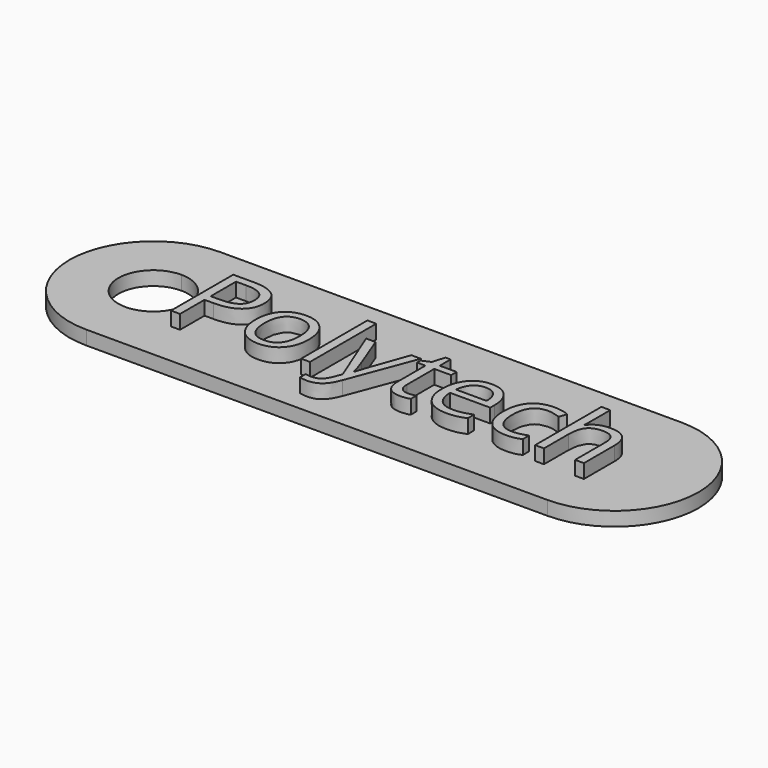
from build123d import *

# Parameters (mm, degrees)
F0_TEXT_SIZE = 7.7975032327
F1_DEPTH     = 2
F0_W         = 0.6323287778
F0_H         = 5.924884097
F2_DEPTH     = 1


# Not quite as in the source:
# - Text() gives the source's letters only with a copy of the font that has no kerning and outlines rounded to 1/6400 em; it was checked with that copy


with BuildPart() as f1:
    # F0 (on Top) → F1 (new body)
    with BuildSketch(Plane.XY):
        with Locations((-13.804265298, -2.749341398)):
            Text('Polytech', F0_TEXT_SIZE, font='Open Sans', text_align=(TextAlign.LEFT, TextAlign.BOTTOM))
    extrude(amount=F1_DEPTH)


with BuildPart() as f2:
    # F0 (on Top) → F2 (new body)
    with BuildSketch(Plane.XY):
        with BuildLine():
            Line((16.5, -0.0275254258), (16.5, 6))
            Line((16.5, 6), (-16.5, 6))
            Line((-16.5, 6), (-16.5, 2.5))
            ThreePointArc((-16.5, 2.5), (-14.732233047, 1.767766953), (-14, 0))
            ThreePointArc((-14, 0), (-14.732233047, -1.767766953), (-16.5, -2.5))
            Line((-16.5, -2.5), (-16.5, -6))
            Line((-16.5, -6), (16.5, -6))
            Line((16.5, -6), (16.5, -2.749341398))
            Line((16.5, -2.749341398), (15.8676712222, -2.749341398))
            Line((15.8676712222, -2.749341398), (15.8676712222, -0.0494559037))
            add(Edge.make_bspline(
                [(15.8676712222, -0.0494559037), (15.8676712222, 0.4598185262), (15.6355736651, 0.7114098415)],
                knots=[0, 0, 0, 1, 1, 1], degree=2))
            add(Edge.make_bspline(
                [(15.6355736651, 0.7114098415), (15.4034761079, 0.9630011567), (14.9076036367, 0.9630011567)],
                knots=[0, 0, 0, 1, 1, 1], degree=2))
            add(Edge.make_bspline(
                [(14.9076036367, 0.9630011567), (14.2496893014, 0.9630011567), (13.9469268712, 0.6048033519)],
                knots=[0, 0, 0, 1, 1, 1], degree=2))
            add(Edge.make_bspline(
                [(13.9469268712, 0.6048033519), (13.644164441, 0.2466055472), (13.644164441, -0.5672588527)],
                knots=[0, 0, 0, 1, 1, 1], degree=2))
            Line((13.644164441, -0.5672588527), (13.644164441, -2.749341398))
            Line((13.644164441, -2.749341398), (13.0118356632, -2.749341398))
            Line((13.0118356632, -2.749341398), (13.0118356632, 3.175542699))
            Line((13.0118356632, 3.175542699), (13.644164441, 3.175542699))
            Line((13.644164441, 3.175542699), (13.644164441, 1.3821169555))
            add(Edge.make_bspline(
                [(13.644164441, 1.3821169555), (13.644164441, 1.0580332273), (13.613705444, 0.8448202483)],
                knots=[0, 0, 0, 1, 1, 1], degree=2))
            Line((13.613705444, 0.8448202483), (13.6514746003, 0.8448202483))
            add(Edge.make_bspline(
                [(13.6514746003, 0.8448202483), (13.837883662, 1.1457551387), (14.182679508, 1.3187622417)],
                knots=[0, 0, 0, 1, 1, 1], degree=2))
            add(Edge.make_bspline(
                [(14.182679508, 1.3187622417), (14.5274753541, 1.4917693447), (14.9685216307, 1.4917693447)],
                knots=[0, 0, 0, 1, 1, 1], degree=2))
            add(Edge.make_bspline(
                [(14.9685216307, 1.4917693447), (15.7336516354, 1.4917693447), (16.1168258177, 1.1280889205)],
                knots=[0, 0, 0, 1, 1, 1], degree=2))
            add(Edge.make_bspline(
                [(16.1168258177, 1.1280889205), (16.5, 0.7644084962), (16.5, -0.0275254258)],
                knots=[0, 0, 0, 1, 1, 1], degree=2))
        make_face()
        with BuildLine():
            Line((-0.7361372239, -2.7724902357), (-2.4199105782, 1.4235411914))
            Line((-2.4199105782, 1.4235411914), (-1.741284125, 1.4235411914))
            Line((-1.741284125, 1.4235411914), (-0.8275142149, -0.9559156545))
            add(Edge.make_bspline(
                [(-0.8275142149, -0.9559156545), (-0.5277976844, -1.7709984143), (-0.4546960916, -2.1328512987)],
                knots=[0, 0, 0, 1, 1, 1], degree=2))
            Line((-0.4546960916, -2.1328512987), (-0.4242370946, -2.1328512987))
            add(Edge.make_bspline(
                [(-0.4242370946, -2.1328512987), (-0.3755026994, -1.9379137179), (-0.217115915, -1.4676268041)],
                knots=[0, 0, 0, 1, 1, 1], degree=2))
            add(Edge.make_bspline(
                [(-0.217115915, -1.4676268041), (-0.0587291306, -0.9973398904), (0.8172716232, 1.4235411914)],
                knots=[0, 0, 0, 1, 1, 1], degree=2))
            Line((0.8172716232, 1.4235411914), (1.4946797165, 1.4235411914))
            Line((1.4946797165, 1.4235411914), (-0.298746027, -3.3280623411))
            add(Edge.make_bspline(
                [(-0.298746027, -3.3280623411), (-0.5655668407, -4.0322743518), (-0.9213279257, -4.3277266227)],
                knots=[0, 0, 0, 1, 1, 1], degree=2))
            add(Edge.make_bspline(
                [(-0.9213279257, -4.3277266227), (-1.2770890107, -4.6231788936), (-1.7948919598, -4.6231788936)],
                knots=[0, 0, 0, 1, 1, 1], degree=2))
            add(Edge.make_bspline(
                [(-1.7948919598, -4.6231788936), (-2.0848616112, -4.6231788936), (-2.3663027435, -4.5573874601)],
                knots=[0, 0, 0, 1, 1, 1], degree=2))
            Line((-2.3663027435, -4.5573874601), (-2.3663027435, -4.0517681098))
            add(Edge.make_bspline(
                [(-2.3663027435, -4.0517681098), (-2.1567448441, -4.0968474254), (-1.8984525496, -4.0968474254)],
                knots=[0, 0, 0, 1, 1, 1], degree=2))
            add(Edge.make_bspline(
                [(-1.8984525496, -4.0968474254), (-1.2466300137, -4.0968474254), (-0.968843961, -3.3658314973)],
                knots=[0, 0, 0, 1, 1, 1], degree=2))
            Line((-0.968843961, -3.3658314973), (-0.7361372239, -2.7724902357))
        make_face(mode=Mode.SUBTRACT)
        with BuildLine():
            add(Edge.make_bspline(
                [(-5.3543303495, 0.9173126612), (-4.8383549403, 0.3343274586), (-4.8383549403, -0.6586358437)],
                knots=[0, 0, 0, 1, 1, 1], degree=2))
            add(Edge.make_bspline(
                [(-4.8383549403, -0.6586358437), (-4.8383549403, -1.6796214233), (-5.3518936297, -2.2528597469)],
                knots=[0, 0, 0, 1, 1, 1], degree=2))
            add(Edge.make_bspline(
                [(-5.3518936297, -2.2528597469), (-5.8654323192, -2.8260980705), (-6.77189207, -2.8260980705)],
                knots=[0, 0, 0, 1, 1, 1], degree=2))
            add(Edge.make_bspline(
                [(-6.77189207, -2.8260980705), (-7.3323376149, -2.8260980705), (-7.7660737322, -2.5629323363)],
                knots=[0, 0, 0, 1, 1, 1], degree=2))
            add(Edge.make_bspline(
                [(-7.7660737322, -2.5629323363), (-8.1998098495, -2.2997666022), (-8.4361716662, -1.8087675706)],
                knots=[0, 0, 0, 1, 1, 1], degree=2))
            add(Edge.make_bspline(
                [(-8.4361716662, -1.8087675706), (-8.672533483, -1.3177685389), (-8.672533483, -0.6586358437)],
                knots=[0, 0, 0, 1, 1, 1], degree=2))
            add(Edge.make_bspline(
                [(-8.672533483, -0.6586358437), (-8.672533483, 0.3611313759), (-8.1620406932, 0.9307146199)],
                knots=[0, 0, 0, 1, 1, 1], degree=2))
            add(Edge.make_bspline(
                [(-8.1620406932, 0.9307146199), (-7.6515479034, 1.5002978638), (-6.7450881526, 1.5002978638)],
                knots=[0, 0, 0, 1, 1, 1], degree=2))
            add(Edge.make_bspline(
                [(-6.7450881526, 1.5002978638), (-5.8703057587, 1.5002978638), (-5.3543303495, 0.9173126612)],
                knots=[0, 0, 0, 1, 1, 1], degree=2))
        make_face(mode=Mode.SUBTRACT)
        with BuildLine():
            add(Edge.make_bspline(
                [(3.0285948056, -2.1017831217), (3.207693708, -2.3034216819), (3.5195938373, -2.3034216819)],
                knots=[0, 0, 0, 1, 1, 1], degree=2))
            add(Edge.make_bspline(
                [(3.5195938373, -2.3034216819), (3.6877275007, -2.3034216819), (3.8436775654, -2.2790544843)],
                knots=[0, 0, 0, 1, 1, 1], degree=2))
            add(Edge.make_bspline(
                [(3.8436775654, -2.2790544843), (3.9996276301, -2.2546872867), (4.0910046211, -2.2278833693)],
                knots=[0, 0, 0, 1, 1, 1], degree=2))
            Line((4.0910046211, -2.2278833693), (4.0910046211, -2.7115722417))
            add(Edge.make_bspline(
                [(4.0910046211, -2.7115722417), (3.9886623911, -2.7603066369), (3.7888513708, -2.7932023537)],
                knots=[0, 0, 0, 1, 1, 1], degree=2))
            add(Edge.make_bspline(
                [(3.7888513708, -2.7932023537), (3.5890403505, -2.8260980705), (3.4282168463, -2.8260980705)],
                knots=[0, 0, 0, 1, 1, 1], degree=2))
            add(Edge.make_bspline(
                [(3.4282168463, -2.8260980705), (2.2183854853, -2.8260980705), (2.2183854853, -1.550475276)],
                knots=[0, 0, 0, 1, 1, 1], degree=2))
            Line((2.2183854853, -1.550475276), (2.2183854853, 0.9325421597))
            Line((2.2183854853, 0.9325421597), (1.6201707842, 0.9325421597))
            Line((1.6201707842, 0.9325421597), (1.6201707842, 1.2371321297))
            Line((1.6201707842, 1.2371321297), (2.2183854853, 1.5002978638))
            Line((2.2183854853, 1.5002978638), (2.4839879392, 2.3909189362))
            Line((2.4839879392, 2.3909189362), (2.8494959032, 2.3909189362))
            Line((2.8494959032, 2.3909189362), (2.8494959032, 1.4235411914))
            Line((2.8494959032, 1.4235411914), (4.0605456241, 1.4235411914))
            Line((4.0605456241, 1.4235411914), (4.0605456241, 0.9325421597))
            Line((4.0605456241, 0.9325421597), (2.8494959032, 0.9325421597))
            Line((2.8494959032, 0.9325421597), (2.8494959032, -1.5236713586))
            add(Edge.make_bspline(
                [(2.8494959032, -1.5236713586), (2.8494959032, -1.9001445616), (3.0285948056, -2.1017831217)],
                knots=[0, 0, 0, 1, 1, 1], degree=2))
        make_face(mode=Mode.SUBTRACT)
        with BuildLine():
            add(Edge.make_bspline(
                [(7.4085985746, -2.7627433567), (7.110100404, -2.8260980705), (6.6873295256, -2.8260980705)],
                knots=[0, 0, 0, 1, 1, 1], degree=2))
            add(Edge.make_bspline(
                [(6.6873295256, -2.8260980705), (5.7625943766, -2.8260980705), (5.2271252093, -2.261997446)],
                knots=[0, 0, 0, 1, 1, 1], degree=2))
            add(Edge.make_bspline(
                [(5.2271252093, -2.261997446), (4.691656042, -1.6978968215), (4.691656042, -0.6976233599)],
                knots=[0, 0, 0, 1, 1, 1], degree=2))
            add(Edge.make_bspline(
                [(4.691656042, -0.6976233599), (4.691656042, 0.3123969807), (5.188746873, 0.9063474223)],
                knots=[0, 0, 0, 1, 1, 1], degree=2))
            add(Edge.make_bspline(
                [(5.188746873, 0.9063474223), (5.6858377041, 1.5002978638), (6.5240693016, 1.5002978638)],
                knots=[0, 0, 0, 1, 1, 1], degree=2))
            add(Edge.make_bspline(
                [(6.5240693016, 1.5002978638), (7.3074747046, 1.5002978638), (7.7643596596, 0.9843224546)],
                knots=[0, 0, 0, 1, 1, 1], degree=2))
            add(Edge.make_bspline(
                [(7.7643596596, 0.9843224546), (8.2212446146, 0.4683470454), (8.2212446146, -0.3771947114)],
                knots=[0, 0, 0, 1, 1, 1], degree=2))
            Line((8.2212446146, -0.3771947114), (8.2212446146, -0.7768167521))
            Line((8.2212446146, -0.7768167521), (5.3471336575, -0.7768167521))
            add(Edge.make_bspline(
                [(5.3471336575, -0.7768167521), (5.3666274155, -1.5114877598), (5.7187334209, -1.8922252223)],
                knots=[0, 0, 0, 1, 1, 1], degree=2))
            add(Edge.make_bspline(
                [(5.7187334209, -1.8922252223), (6.0708394262, -2.2729626849), (6.7104783633, -2.2729626849)],
                knots=[0, 0, 0, 1, 1, 1], degree=2))
            add(Edge.make_bspline(
                [(6.7104783633, -2.2729626849), (7.384231377, -2.2729626849), (8.0421457123, -1.9915215526)],
                knots=[0, 0, 0, 1, 1, 1], degree=2))
            Line((8.0421457123, -1.9915215526), (8.0421457123, -2.5556221771))
            add(Edge.make_bspline(
                [(8.0421457123, -2.5556221771), (7.7070967452, -2.6993886429), (7.4085985746, -2.7627433567)],
                knots=[0, 0, 0, 1, 1, 1], degree=2))
        make_face(mode=Mode.SUBTRACT)
        with BuildLine():
            add(Edge.make_bspline(
                [(12.0213090807, -2.6080116519), (11.6034116418, -2.8260980705), (10.9674277844, -2.8260980705)],
                knots=[0, 0, 0, 1, 1, 1], degree=2))
            add(Edge.make_bspline(
                [(10.9674277844, -2.8260980705), (10.0609680336, -2.8260980705), (9.5638772025, -2.2680892454)],
                knots=[0, 0, 0, 1, 1, 1], degree=2))
            add(Edge.make_bspline(
                [(9.5638772025, -2.2680892454), (9.0667863714, -1.7100804203), (9.0667863714, -0.6890948407)],
                knots=[0, 0, 0, 1, 1, 1], degree=2))
            add(Edge.make_bspline(
                [(9.0667863714, -0.6890948407), (9.0667863714, 0.3574762963), (9.5717965417, 0.9288870801)],
                knots=[0, 0, 0, 1, 1, 1], degree=2))
            add(Edge.make_bspline(
                [(9.5717965417, 0.9288870801), (10.0768067121, 1.5002978638), (11.0088520203, 1.5002978638)],
                knots=[0, 0, 0, 1, 1, 1], degree=2))
            add(Edge.make_bspline(
                [(11.0088520203, 1.5002978638), (11.3097869107, 1.5002978638), (11.6107218011, 1.4351156102)],
                knots=[0, 0, 0, 1, 1, 1], degree=2))
            add(Edge.make_bspline(
                [(11.6107218011, 1.4351156102), (11.9116566915, 1.3699333567), (12.0822270747, 1.2822114453)],
                knots=[0, 0, 0, 1, 1, 1], degree=2))
            Line((12.0822270747, 1.2822114453), (11.8885078538, 0.746133098))
            add(Edge.make_bspline(
                [(11.8885078538, 0.746133098), (11.6789499544, 0.8301999298), (11.4316228987, 0.8850261244)],
                knots=[0, 0, 0, 1, 1, 1], degree=2))
            add(Edge.make_bspline(
                [(11.4316228987, 0.8850261244), (11.1842958431, 0.939852319), (10.9942317018, 0.939852319)],
                knots=[0, 0, 0, 1, 1, 1], degree=2))
            add(Edge.make_bspline(
                [(10.9942317018, 0.939852319), (9.7222639869, 0.939852319), (9.7222639869, -0.6817846815)],
                knots=[0, 0, 0, 1, 1, 1], degree=2))
            add(Edge.make_bspline(
                [(9.7222639869, -0.6817846815), (9.7222639869, -1.4505697658), (10.0323365764, -1.8617662253)],
                knots=[0, 0, 0, 1, 1, 1], degree=2))
            add(Edge.make_bspline(
                [(10.0323365764, -1.8617662253), (10.3424091659, -2.2729626849), (10.951589106, -2.2729626849)],
                knots=[0, 0, 0, 1, 1, 1], degree=2))
            add(Edge.make_bspline(
                [(10.951589106, -2.2729626849), (11.4730471347, -2.2729626849), (12.0213090807, -2.0487844669)],
                knots=[0, 0, 0, 1, 1, 1], degree=2))
            Line((12.0213090807, -2.0487844669), (12.0213090807, -2.6080116519))
        make_face(mode=Mode.SUBTRACT)
        with BuildLine():
            add(Edge.make_bspline(
                [(-11.5953788354, 2.8173448942), (-9.5095467206, 2.8173448942), (-9.5095467206, 1.1957078938)],
                knots=[0, 0, 0, 1, 1, 1], degree=2))
            add(Edge.make_bspline(
                [(-9.5095467206, 1.1957078938), (-9.5095467206, 0.350166137), (-10.0864401238, -0.1048912782)],
                knots=[0, 0, 0, 1, 1, 1], degree=2))
            add(Edge.make_bspline(
                [(-10.0864401238, -0.1048912782), (-10.6633335271, -0.5599486934), (-11.7367085815, -0.5599486934)],
                knots=[0, 0, 0, 1, 1, 1], degree=2))
            Line((-11.7367085815, -0.5599486934), (-12.392186197, -0.5599486934))
            Line((-12.392186197, -0.5599486934), (-12.392186197, -2.749341398))
            Line((-12.392186197, -2.749341398), (-13.0391352933, -2.749341398))
            Line((-13.0391352933, -2.749341398), (-13.0391352933, 2.8173448942))
            Line((-13.0391352933, 2.8173448942), (-11.5953788354, 2.8173448942))
        make_face(mode=Mode.SUBTRACT)
        with Locations((-3.4134830605, 0.2131006505)):
            Rectangle(F0_W, F0_H, mode=Mode.SUBTRACT)
        with BuildLine():
            ThreePointArc((16.5, -6), (22.5, 0), (16.5, 6))
            Line((16.5, 6), (16.5, -0.0275254258))
            Line((16.5, -0.0275254258), (16.5, -2.749341398))
            Line((16.5, -2.749341398), (16.5, -6))
        make_face()
        with BuildLine():
            Line((-16.5, 2.5), (-16.5, 6))
            ThreePointArc((-16.5, 6), (-22.5, 0), (-16.5, -6))
            Line((-16.5, -6), (-16.5, -2.5))
            ThreePointArc((-16.5, -2.5), (-19, 0), (-16.5, 2.5))
        make_face()
    extrude(amount=F2_DEPTH)


with BuildPart() as f2b:
    # F0 (on Top) → F2, piece 2 (new body)
    with BuildSketch(Plane.XY):
        with BuildLine():
            Line((-12.392186197, 2.2568993494), (-12.392186197, -0.0043765881))
            Line((-12.392186197, -0.0043765881), (-11.8085918144, -0.0043765881))
            add(Edge.make_bspline(
                [(-11.8085918144, -0.0043765881), (-10.948429739, -0.0043765881), (-10.5640371969, 0.2734094646)],
                knots=[0, 0, 0, 1, 1, 1], degree=2))
            add(Edge.make_bspline(
                [(-10.5640371969, 0.2734094646), (-10.1796446547, 0.5511955172), (-10.1796446547, 1.1652488968)],
                knots=[0, 0, 0, 1, 1, 1], degree=2))
            add(Edge.make_bspline(
                [(-10.1796446547, 1.1652488968), (-10.1796446547, 1.7171659225), (-10.5414975391, 1.9870326359)],
                knots=[0, 0, 0, 1, 1, 1], degree=2))
            add(Edge.make_bspline(
                [(-10.5414975391, 1.9870326359), (-10.9033504235, 2.2568993494), (-11.6684804282, 2.2568993494)],
                knots=[0, 0, 0, 1, 1, 1], degree=2))
            Line((-11.6684804282, 2.2568993494), (-12.392186197, 2.2568993494))
        make_face()
    extrude(amount=F2_DEPTH)


with BuildPart() as f2c:
    # F0 (on Top) → F2, piece 3 (new body)
    with BuildSketch(Plane.XY):
        with BuildLine():
            add(Edge.make_bspline(
                [(-7.7008914786, 0.5554597768), (-8.0170558675, 0.1479183969), (-8.0170558675, -0.6586358437)],
                knots=[0, 0, 0, 1, 1, 1], degree=2))
            add(Edge.make_bspline(
                [(-8.0170558675, -0.6586358437), (-8.0170558675, -1.459098285), (-7.697236399, -1.8776049038)],
                knots=[0, 0, 0, 1, 1, 1], degree=2))
            add(Edge.make_bspline(
                [(-7.697236399, -1.8776049038), (-7.3774169304, -2.2961115226), (-6.7572717514, -2.2961115226)],
                knots=[0, 0, 0, 1, 1, 1], degree=2))
            add(Edge.make_bspline(
                [(-6.7572717514, -2.2961115226), (-6.1359082126, -2.2961115226), (-5.8142612042, -1.8794324436)],
                knots=[0, 0, 0, 1, 1, 1], degree=2))
            add(Edge.make_bspline(
                [(-5.8142612042, -1.8794324436), (-5.4926141959, -1.4627533646), (-5.4926141959, -0.6586358437)],
                knots=[0, 0, 0, 1, 1, 1], degree=2))
            add(Edge.make_bspline(
                [(-5.4926141959, -0.6586358437), (-5.4926141959, 0.136953158), (-5.8142612042, 0.5499771573)],
                knots=[0, 0, 0, 1, 1, 1], degree=2))
            add(Edge.make_bspline(
                [(-5.8142612042, 0.5499771573), (-6.1359082126, 0.9630011567), (-6.7645819107, 0.9630011567)],
                knots=[0, 0, 0, 1, 1, 1], degree=2))
            add(Edge.make_bspline(
                [(-6.7645819107, 0.9630011567), (-7.3847270897, 0.9630011567), (-7.7008914786, 0.5554597768)],
                knots=[0, 0, 0, 1, 1, 1], degree=2))
        make_face()
    extrude(amount=F2_DEPTH)


with BuildPart() as f2d:
    # F0 (on Top) → F2, piece 4 (new body)
    with BuildSketch(Plane.XY):
        with BuildLine():
            add(Edge.make_bspline(
                [(7.2776248875, 0.6523193873), (7.0114132537, 0.970311316), (6.5155407825, 0.970311316)],
                knots=[0, 0, 0, 1, 1, 1], degree=2))
            add(Edge.make_bspline(
                [(6.5155407825, 0.970311316), (6.0135765119, 0.970311316), (5.7144691613, 0.6431816882)],
                knots=[0, 0, 0, 1, 1, 1], degree=2))
            add(Edge.make_bspline(
                [(5.7144691613, 0.6431816882), (5.4153618107, 0.3160520604), (5.361753976, -0.2626688827)],
                knots=[0, 0, 0, 1, 1, 1], degree=2))
            Line((5.361753976, -0.2626688827), (7.5438365213, -0.2626688827))
            add(Edge.make_bspline(
                [(7.5438365213, -0.2626688827), (7.5438365213, 0.3343274586), (7.2776248875, 0.6523193873)],
                knots=[0, 0, 0, 1, 1, 1], degree=2))
        make_face()
    extrude(amount=F2_DEPTH)


solid = Compound([f1.part, f2.part, f2b.part, f2c.part, f2d.part])
